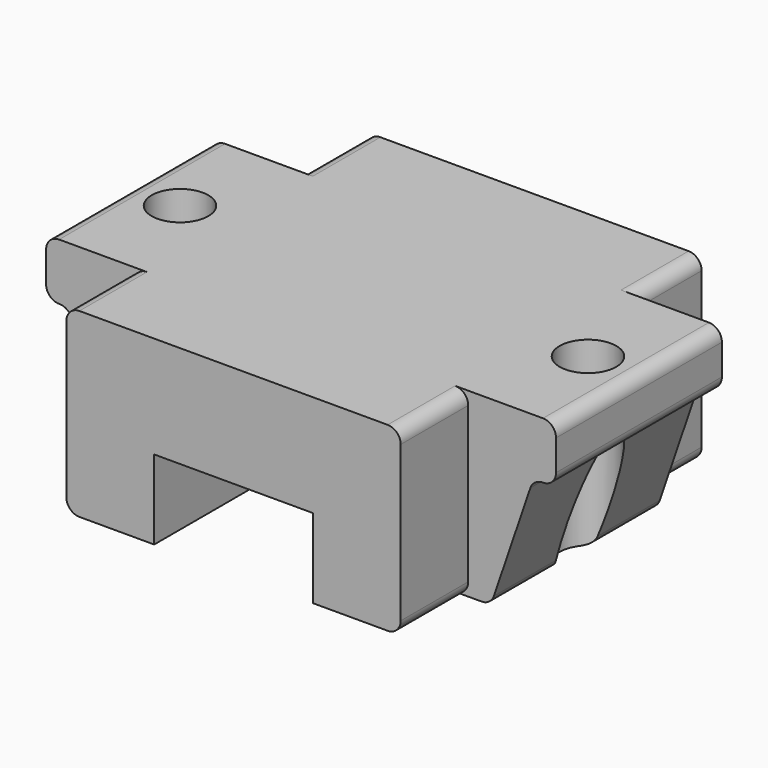
from build123d import *

# Parameters (mm, degrees)
F1_DEPTH      = 36.6
F3_DEPTH      = 14.9
F3_DEPTH_BACK = 51.5
F4_R          = 5
F5_DEPTH      = 32.001
F6_T4_DEPTH   = 18.3
F6_S5_R       = 5
F6_T6_DEPTH   = 11
F6_T10_DEPTH  = 18.3
F6_S11_R      = 5
F6_T12_DEPTH  = 11
F6_T16_DEPTH  = 18.3
F6_S17_R      = 5
F6_T18_DEPTH  = 11
F6_T22_DEPTH  = 18.3
F6_S23_R      = 5
F6_T24_DEPTH  = 11
F6_T25_DEPTH  = 48.1
F6_T27_DEPTH  = 22.1993140666
F6_T29_DEPTH  = 22.1993140666
F6_T31_DEPTH  = 20.65
F6_T33_DEPTH  = 20.65


# Not quite as in the source:
# - a fillet or chamfer that OpenCascade refuses, or shapes differently, is made with other operations: its cross-section is extruded or revolved along the edge and cut away or added


with BuildPart() as f1:
    # F0 (on Front) → F1 (new body)
    with BuildSketch(Plane.XZ):
        Polygon((-28.4127721637, 8.7557665049), (-43.9127721637, 8.7557665049), (-43.9127721637, -1.2442334951), (-39.9127721637, -1.2442334951), (-32.4127721637, -23.2442334951), (-28.4127721637, -23.2442334951), align=None)
        Polygon((30.5872278363, 8.7557665049), (-28.4127721637, 8.7557665049), (-28.4127721637, -23.2442334951), (-12.9127721637, -23.2442334951), (-12.9127721637, -9.2442334951), (15.0872278363, -9.2442334951), (15.0872278363, -23.2442334951), (30.5872278363, -23.2442334951), align=None)
        Polygon((46.0872278363, 8.7557665049), (30.5872278363, 8.7557665049), (30.5872278363, -23.2442334951), (34.5872278363, -23.2442334951), (42.0872278363, -1.2442334951), (46.0872278363, -1.2442334951), align=None)
    extrude(amount=F1_DEPTH)

    # F2 (on face) → F3 (join, two sides)
    with BuildSketch(Plane(origin=(0, 0, 0), x_dir=(-1, 0, 0), z_dir=(0, 1, 0))) as f3_sk:
        Polygon((28.4127721637, 8.7557665049), (-30.5872278363, 8.7557665049), (-30.5872278363, -23.2442334951), (-15.0872278363, -23.2442334951), (-15.0872278363, -9.2442334951), (12.9127721637, -9.2442334951), (12.9127721637, -23.2442334951), (28.4127721637, -23.2442334951), align=None)
    extrude(amount=F3_DEPTH)
    extrude(f3_sk.sketch, amount=-F3_DEPTH_BACK)

    # F4 (on face) → F5 (cut, through all)
    with BuildSketch(Plane.XY.offset(8.7557665049)):
        with Locations((-34.9127721637, -18.3)):
            Circle(F4_R)
        with Locations((37.0872278363, -18.3)):
            Circle(F4_R)
    extrude(amount=-F5_DEPTH, mode=Mode.SUBTRACT)

    # F6: fillet of radius 2.3 on 20 edges, made by hand


with BuildPart() as f6_tool2:
    # F6_s3 → F6_t4 (new body)
    with BuildSketch(Plane.XZ.offset(18.3)):
        with BuildLine():
            ThreePointArc((-41.5586603808, -1.2442334951), (-40.2201808476, -1.6738130774), (-39.381686948, -2.8020834612))
            Line((-39.381686948, -2.8020834612), (-39.9127721637, -1.2442334951))
            Line((-39.9127721637, -1.2442334951), (-41.5586603808, -1.2442334951))
        make_face()
    extrude(amount=F6_T4_DEPTH)

    # F6_s5 → F6_t6 (cut, symmetric)
    with BuildSketch(Plane.XY.offset(-2)):
        with Locations((-34.9127721637, -18.3)):
            Circle(F6_S5_R)
    extrude(amount=F6_T6_DEPTH, both=True, mode=Mode.SUBTRACT)


with BuildPart() as f1_1:
    add(f1.part)

    # F6_t1: union F6_tool2
    add(f6_tool2.part)


with BuildPart() as f6_tool8:
    # F6_s9 → F6_t10 (new body)
    with BuildSketch(Plane.XZ.offset(18.3)):
        with BuildLine():
            ThreePointArc((43.7331160534, -1.2442334951), (42.3946365201, -1.6738130774), (41.5561426205, -2.8020834612))
            Line((41.5561426205, -2.8020834612), (42.0872278363, -1.2442334951))
            Line((42.0872278363, -1.2442334951), (43.7331160534, -1.2442334951))
        make_face()
    extrude(amount=F6_T10_DEPTH)

    # F6_s11 → F6_t12 (cut, symmetric)
    with BuildSketch(Plane.XY.offset(-2)):
        with Locations((37.0872278363, -18.3)):
            Circle(F6_S11_R)
    extrude(amount=F6_T12_DEPTH, both=True, mode=Mode.SUBTRACT)


with BuildPart() as f1_2:
    add(f1_1.part)

    # F6_t7: union F6_tool8
    add(f6_tool8.part)


with BuildPart() as f6_tool14:
    # F6_s15 → F6_t16 (new body)
    with BuildSketch(Plane.XZ):
        with BuildLine():
            ThreePointArc((43.7331160534, -1.2442334951), (42.3946365201, -1.6738130774), (41.5561426205, -2.8020834612))
            Line((41.5561426205, -2.8020834612), (42.0872278363, -1.2442334951))
            Line((42.0872278363, -1.2442334951), (43.7331160534, -1.2442334951))
        make_face()
    extrude(amount=F6_T16_DEPTH)

    # F6_s17 → F6_t18 (cut, symmetric)
    with BuildSketch(Plane.XY.offset(-2)):
        with Locations((37.0872278363, -18.3)):
            Circle(F6_S17_R)
    extrude(amount=F6_T18_DEPTH, both=True, mode=Mode.SUBTRACT)


with BuildPart() as f1_3:
    add(f1_2.part)

    # F6_t13: union F6_tool14
    add(f6_tool14.part)


with BuildPart() as f6_tool20:
    # F6_s21 → F6_t22 (new body)
    with BuildSketch(Plane.XZ):
        with BuildLine():
            ThreePointArc((-41.5586603808, -1.2442334951), (-40.2201808476, -1.6738130774), (-39.381686948, -2.8020834612))
            Line((-39.381686948, -2.8020834612), (-39.9127721637, -1.2442334951))
            Line((-39.9127721637, -1.2442334951), (-41.5586603808, -1.2442334951))
        make_face()
    extrude(amount=F6_T22_DEPTH)

    # F6_s23 → F6_t24 (cut, symmetric)
    with BuildSketch(Plane.XY.offset(-2)):
        with Locations((-34.9127721637, -18.3)):
            Circle(F6_S23_R)
    extrude(amount=F6_T24_DEPTH, both=True, mode=Mode.SUBTRACT)


with BuildPart() as f1_4:
    add(f1_3.part)

    # F6_t19: union F6_tool20
    add(f6_tool20.part)

    # F6_s26 → F6_t25 (cut)
    with BuildSketch(Plane.XZ.offset(-5.75)):
        with BuildLine():
            ThreePointArc((-43.9127721637, 1.0557665049), (-43.2391177605, -0.5705790919), (-41.6127721637, -1.2442334951))
            Line((-41.6127721637, -1.2442334951), (-43.9127721637, -1.2442334951))
            Line((-43.9127721637, -1.2442334951), (-43.9127721637, 1.0557665049))
        make_face()
        with BuildLine():
            ThreePointArc((-43.9127721637, 6.4557665049), (-43.2391177605, 8.0821121016), (-41.6127721637, 8.7557665049))
            Line((-41.6127721637, 8.7557665049), (-43.9127721637, 8.7557665049))
            Line((-43.9127721637, 8.7557665049), (-43.9127721637, 6.4557665049))
        make_face()
        with BuildLine():
            ThreePointArc((46.0872278363, 6.4557665049), (45.413573433, 8.0821121016), (43.7872278363, 8.7557665049))
            Line((43.7872278363, 8.7557665049), (46.0872278363, 8.7557665049))
            Line((46.0872278363, 8.7557665049), (46.0872278363, 6.4557665049))
        make_face()
        with BuildLine():
            ThreePointArc((46.0872278363, 1.0557665049), (45.413573433, -0.5705790919), (43.7872278363, -1.2442334951))
            Line((43.7872278363, -1.2442334951), (46.0872278363, -1.2442334951))
            Line((46.0872278363, -1.2442334951), (46.0872278363, 1.0557665049))
        make_face()
    extrude(amount=F6_T25_DEPTH, mode=Mode.SUBTRACT)

    # F6_s28 → F6_t27 (cut)
    with BuildSketch(Plane.XZ.offset(18.5154064762)):
        with BuildLine():
            ThreePointArc((-30.7668839466, -23.2442334951), (-32.1053634799, -22.8146539129), (-32.9438573795, -21.6863835291))
            Line((-32.9438573795, -21.6863835291), (-32.4127721637, -23.2442334951))
            Line((-32.4127721637, -23.2442334951), (-30.7668839466, -23.2442334951))
        make_face()
        with BuildLine():
            ThreePointArc((35.118313052, -21.6863835291), (34.2798191524, -22.8146539129), (32.9413396192, -23.2442334951))
            Line((32.9413396192, -23.2442334951), (34.5872278363, -23.2442334951))
            Line((34.5872278363, -23.2442334951), (35.118313052, -21.6863835291))
        make_face()
    extrude(amount=F6_T27_DEPTH, mode=Mode.SUBTRACT)

    # F6_s30 → F6_t29 (cut)
    with BuildSketch(Plane.XZ.offset(-4.1147205427)):
        with BuildLine():
            ThreePointArc((-30.7668839466, -23.2442334951), (-32.1053634799, -22.8146539129), (-32.9438573795, -21.6863835291))
            Line((-32.9438573795, -21.6863835291), (-32.4127721637, -23.2442334951))
            Line((-32.4127721637, -23.2442334951), (-30.7668839466, -23.2442334951))
        make_face()
        with BuildLine():
            ThreePointArc((35.118313052, -21.6863835291), (34.2798191524, -22.8146539129), (32.9413396192, -23.2442334951))
            Line((32.9413396192, -23.2442334951), (34.5872278363, -23.2442334951))
            Line((34.5872278363, -23.2442334951), (35.118313052, -21.6863835291))
        make_face()
    extrude(amount=F6_T29_DEPTH, mode=Mode.SUBTRACT)

    # F6_s32 → F6_t31 (cut)
    with BuildSketch(Plane.XZ.offset(36.6)):
        with BuildLine():
            ThreePointArc((-28.4127721637, -20.9442334951), (-27.7391177605, -22.5705790919), (-26.1127721637, -23.2442334951))
            Line((-26.1127721637, -23.2442334951), (-28.4127721637, -23.2442334951))
            Line((-28.4127721637, -23.2442334951), (-28.4127721637, -20.9442334951))
        make_face()
        with BuildLine():
            ThreePointArc((-28.4127721637, 6.4557665049), (-27.7391177605, 8.0821121016), (-26.1127721637, 8.7557665049))
            Line((-26.1127721637, 8.7557665049), (-28.4127721637, 8.7557665049))
            Line((-28.4127721637, 8.7557665049), (-28.4127721637, 6.4557665049))
        make_face()
        with BuildLine():
            ThreePointArc((30.5872278363, 6.4557665049), (29.913573433, 8.0821121016), (28.2872278363, 8.7557665049))
            Line((28.2872278363, 8.7557665049), (30.5872278363, 8.7557665049))
            Line((30.5872278363, 8.7557665049), (30.5872278363, 6.4557665049))
        make_face()
        with BuildLine():
            ThreePointArc((28.2872278363, -23.2442334951), (29.913573433, -22.5705790919), (30.5872278363, -20.9442334951))
            Line((30.5872278363, -20.9442334951), (30.5872278363, -23.2442334951))
            Line((30.5872278363, -23.2442334951), (28.2872278363, -23.2442334951))
        make_face()
    extrude(amount=F6_T31_DEPTH, mode=Mode.SUBTRACT)

    # F6_s34 → F6_t33 (cut)
    with BuildSketch(Plane.XZ.offset(-20.65)):
        with BuildLine():
            ThreePointArc((-28.4127721637, -20.9442334951), (-27.7391177605, -22.5705790919), (-26.1127721637, -23.2442334951))
            Line((-26.1127721637, -23.2442334951), (-28.4127721637, -23.2442334951))
            Line((-28.4127721637, -23.2442334951), (-28.4127721637, -20.9442334951))
        make_face()
        with BuildLine():
            ThreePointArc((-28.4127721637, 6.4557665049), (-27.7391177605, 8.0821121016), (-26.1127721637, 8.7557665049))
            Line((-26.1127721637, 8.7557665049), (-28.4127721637, 8.7557665049))
            Line((-28.4127721637, 8.7557665049), (-28.4127721637, 6.4557665049))
        make_face()
        with BuildLine():
            ThreePointArc((30.5872278363, 6.4557665049), (29.913573433, 8.0821121016), (28.2872278363, 8.7557665049))
            Line((28.2872278363, 8.7557665049), (30.5872278363, 8.7557665049))
            Line((30.5872278363, 8.7557665049), (30.5872278363, 6.4557665049))
        make_face()
        with BuildLine():
            ThreePointArc((30.5872278363, -20.9442334951), (29.913573433, -22.5705790919), (28.2872278363, -23.2442334951))
            Line((28.2872278363, -23.2442334951), (30.5872278363, -23.2442334951))
            Line((30.5872278363, -23.2442334951), (30.5872278363, -20.9442334951))
        make_face()
    extrude(amount=F6_T33_DEPTH, mode=Mode.SUBTRACT)


solid = f1_4.part
